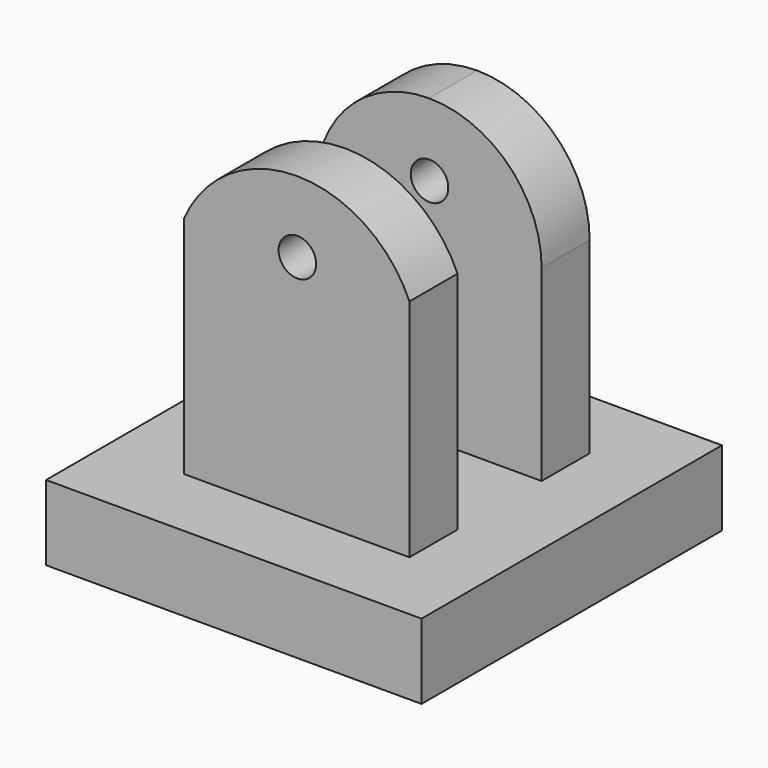
from build123d import *

# Parameters (mm, degrees)
F0_W     = 50
F0_H     = 50
F1_DEPTH = 10
F2_W     = 30
F2_H     = 8
F3_DEPTH = 40
F4_W     = 30
F4_H     = 8
F5_DEPTH = 30
F7_DEPTH = 8
F9_R     = 14.99999
F11_D    = 5


# Not quite as in the source:
# - a fillet or chamfer is up to 0.001 mm smaller than in the source, because OpenCascade refuses the exact size


with BuildPart() as f1:
    # F0 (on Top) → F1 (new body)
    with BuildSketch(Plane.XY):
        with Locations((1.1680293828, -3.1129003775)):
            Rectangle(F0_W, F0_H)
    extrude(amount=F1_DEPTH)

    # F2 (on face) → F3 (join)
    with BuildSketch(Plane.XY.offset(10)):
        with Locations((1.5573729761, 7.8870996225)):
            Rectangle(F2_W, F2_H)
    extrude(amount=F3_DEPTH)

    # F4 (on face) → F5 (join)
    with BuildSketch(Plane.XY.offset(10)):
        with Locations((1.5573729761, -14.1129003775)):
            Rectangle(F4_W, F4_H)
    extrude(amount=F5_DEPTH)

    # F6 (on face) → F7 (join)
    with BuildSketch(Plane.XZ.offset(18.1129003775)):
        with BuildLine():
            Line((-13.4426270239, 40), (16.5573729761, 40))
            ThreePointArc((16.5573729761, 40), (1.5573729761, 49.8339152222), (-13.4426270239, 40))
        make_face()
    extrude(amount=-F7_DEPTH)

    # F9 (radius 15 in the source; OpenCascade refuses exactly that, so slightly less here)
    f9_edges = [f1.edges().sort_by_distance(p)[0] for p in [
        (16.557373, 7.8871, 50),
        (-13.442627, 7.8871, 50),
    ]]
    fillet(f9_edges, radius=F9_R)

    # F11 (through all)
    with Locations(Plane.XZ.offset(18.1129003775)):
        with Locations((1.6286504688, 40.3330288827)):
            Hole(F11_D / 2)


solid = f1.part
